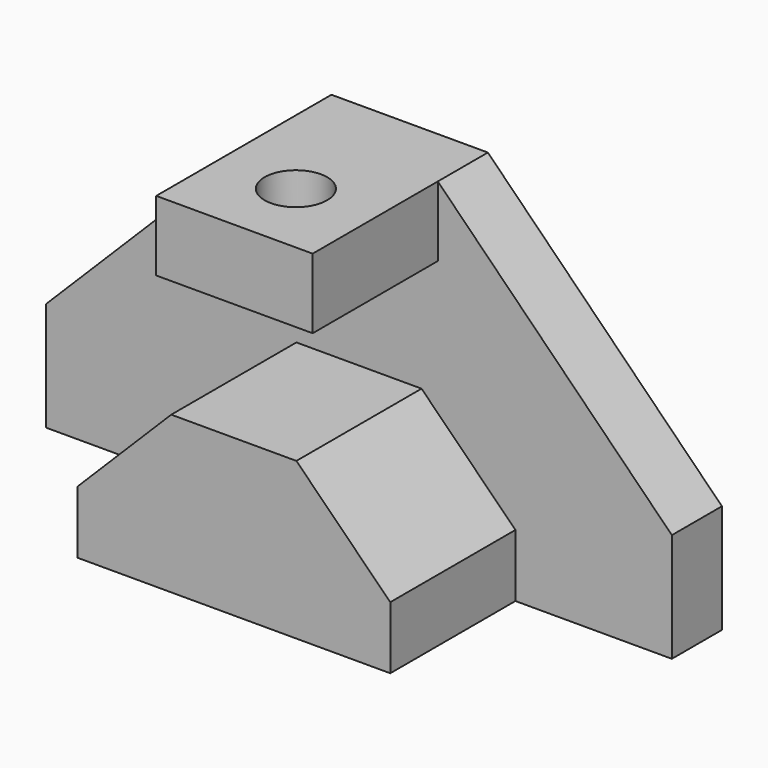
from build123d import *

# Parameters (mm, degrees)
F1_DEPTH      = 31.75
F2_DEPTH      = 12.7
F0_W          = 31.75
F0_H          = 14.224
F3_DEPTH      = 31.75
F3_DEPTH_BACK = 12.7
F4_DEPTH      = 12.7
F5_R          = 6.35
F6_DEPTH      = 14.224


with BuildPart() as f1:
    # F0 (on Front) → F1 (new body)
    with BuildSketch(Plane.XZ):
        Polygon((-19.05, 0), (0, 0), (25.4, 0), (44.45, 0), (44.45, 12.7), (25.4, 31.75), (0, 31.75), (-19.05, 12.7), align=None)
    extrude(amount=F1_DEPTH)


with BuildPart() as f2:
    # F0 (on Front) → F2 (new body)
    with BuildSketch(Plane.XZ):
        Polygon((-50.8, 0), (-19.05, 0), (-19.05, 12.7), (0, 31.75), (25.4, 31.75), (44.45, 12.7), (44.45, 0), (76.2, 0), (76.2, 22.098), (28.702, 69.85), (28.702, 55.626), (-3.048, 55.626), (-3.048, 69.85), (-50.8, 22.098), align=None)
    extrude(amount=-F2_DEPTH)

    # F0 (on Front) → F3 (join, two sides)
    with BuildSketch(Plane.XZ) as f3_sk:
        with Locations((12.827, 62.738)):
            Rectangle(F0_W, F0_H)
    extrude(amount=F3_DEPTH)
    extrude(f3_sk.sketch, amount=-F3_DEPTH_BACK)

    # F4 (add, through all): a face of the model
    f4_faces = [f1.part.faces().sort_by_distance(p)[0] for p in [
        (12.7, 0, 13.7841463415),
    ]]
    extrude(f4_faces, amount=F4_DEPTH)

    # F5 (on face) → F6 (cut)
    with BuildSketch(Plane.XY.offset(69.85)):
        with Locations((12.7, -16.002)):
            Circle(F5_R)
    extrude(amount=-F6_DEPTH, mode=Mode.SUBTRACT)


solid = Compound([f1.part, f2.part])
